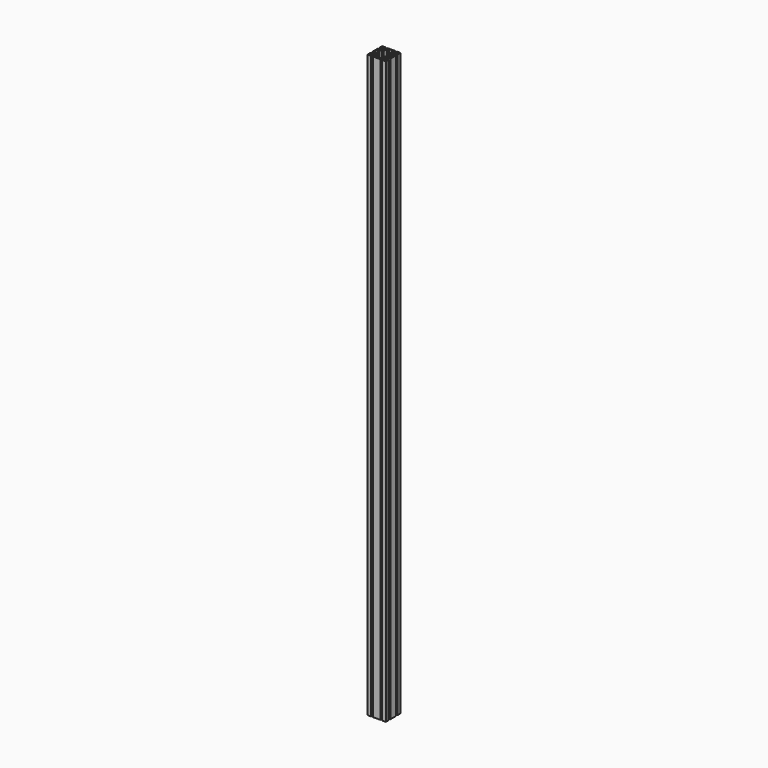
from build123d import *

# Parameters (mm, degrees)
F0_R     = 3
F0_R_2   = 2.5
F1_DEPTH = 1900
F2_R     = 2
F3_R     = 7


# Not quite as in the source:
# - a feature names something its author has since deleted; it is built from what else it names


with BuildPart() as f1:
    # F0 (on Top) → F1 (new body)
    with BuildSketch(Plane.XY):
        with BuildLine():
            Line((18.15, -30), (30, -30))
            Line((30, -30), (30, -18.15))
            Line((30, -18.15), (27.5, -18.15))
            Line((27.5, -18.15), (27.5, -20.15))
            Line((27.5, -20.15), (21.5477069044, -20.15))
            ThreePointArc((21.5477069044, -20.15), (19.5, -15), (21.5477069044, -9.85))
            Line((21.5477069044, -9.85), (27.5, -9.85))
            Line((27.5, -9.85), (27.5, -11.85))
            Line((27.5, -11.85), (30, -11.85))
            Line((30, -11.85), (30, 11.85))
            Line((30, 11.85), (27.5, 11.85))
            Line((27.5, 11.85), (27.5, 9.85))
            Line((27.5, 9.85), (21.5477069044, 9.85))
            ThreePointArc((21.5477069044, 9.85), (19.5, 15), (21.5477069044, 20.15))
            Line((21.5477069044, 20.15), (27.5, 20.15))
            Line((27.5, 20.15), (27.5, 18.15))
            Line((27.5, 18.15), (30, 18.15))
            Line((30, 18.15), (30, 30))
            Line((30, 30), (18.15, 30))
            Line((18.15, 30), (18.15, 27.5))
            Line((18.15, 27.5), (20.15, 27.5))
            Line((20.15, 27.5), (20.15, 21.5477069044))
            ThreePointArc((20.15, 21.5477069044), (15, 19.5), (9.85, 21.5477069044))
            Line((9.85, 21.5477069044), (9.85, 27.5))
            Line((9.85, 27.5), (11.85, 27.5))
            Line((11.85, 27.5), (11.85, 30))
            Line((11.85, 30), (-11.85, 30))
            Line((-11.85, 30), (-11.85, 27.5))
            Line((-11.85, 27.5), (-9.85, 27.5))
            Line((-9.85, 27.5), (-9.85, 21.5477069044))
            ThreePointArc((-9.85, 21.5477069044), (-15, 19.5), (-20.15, 21.5477069044))
            Line((-20.15, 21.5477069044), (-20.15, 27.5))
            Line((-20.15, 27.5), (-18.15, 27.5))
            Line((-18.15, 27.5), (-18.15, 30))
            Line((-18.15, 30), (-30, 30))
            Line((-30, 30), (-30, 18.15))
            Line((-30, 18.15), (-27.5, 18.15))
            Line((-27.5, 18.15), (-27.5, 20.15))
            Line((-27.5, 20.15), (-21.5477069044, 20.15))
            ThreePointArc((-21.5477069044, 20.15), (-19.5, 15), (-21.5477069044, 9.85))
            Line((-21.5477069044, 9.85), (-27.5, 9.85))
            Line((-27.5, 9.85), (-27.5, 11.85))
            Line((-27.5, 11.85), (-30, 11.85))
            Line((-30, 11.85), (-30, -11.85))
            Line((-30, -11.85), (-27.5, -11.85))
            Line((-27.5, -11.85), (-27.5, -9.85))
            Line((-27.5, -9.85), (-21.5477069044, -9.85))
            ThreePointArc((-21.5477069044, -9.85), (-19.5, -15), (-21.5477069044, -20.15))
            Line((-21.5477069044, -20.15), (-27.5, -20.15))
            Line((-27.5, -20.15), (-27.5, -18.15))
            Line((-27.5, -18.15), (-30, -18.15))
            Line((-30, -18.15), (-30, -30))
            Line((-30, -30), (-18.15, -30))
            Line((-18.15, -30), (-18.15, -27.5))
            Line((-18.15, -27.5), (-20.15, -27.5))
            Line((-20.15, -27.5), (-20.15, -21.5477069044))
            ThreePointArc((-20.15, -21.5477069044), (-15, -19.5), (-9.85, -21.5477069044))
            Line((-9.85, -21.5477069044), (-9.85, -27.5))
            Line((-9.85, -27.5), (-11.85, -27.5))
            Line((-11.85, -27.5), (-11.85, -30))
            Line((-11.85, -30), (11.85, -30))
            Line((11.85, -30), (11.85, -27.5))
            Line((11.85, -27.5), (9.85, -27.5))
            Line((9.85, -27.5), (9.85, -21.5477069044))
            ThreePointArc((9.85, -21.5477069044), (15, -19.5), (20.15, -21.5477069044))
            Line((20.15, -21.5477069044), (20.15, -27.5))
            Line((20.15, -27.5), (18.15, -27.5))
            Line((18.15, -27.5), (18.15, -30))
        make_face()
        with Locations((-25, -25)):
            Circle(F0_R, mode=Mode.SUBTRACT)
        with Locations((-15, -15)):
            Circle(F0_R_2, mode=Mode.SUBTRACT)
        with Locations((25, -25)):
            Circle(F0_R, mode=Mode.SUBTRACT)
        with Locations((15, -15)):
            Circle(F0_R_2, mode=Mode.SUBTRACT)
        with Locations((-25, 25)):
            Circle(F0_R, mode=Mode.SUBTRACT)
        with Locations((-15, 15)):
            Circle(F0_R_2, mode=Mode.SUBTRACT)
        Polygon((-7, 22), (-7, 27.5), (0, 27.5), (7, 27.5), (7, 22), (10, 16), (10, 10), (16, 10), (22, 7), (27.5, 7), (27.5, 0), (27.5, -7), (22, -7), (16, -10), (10, -10), (10, -16), (7, -22), (7, -27.5), (0, -27.5), (-7, -27.5), (-7, -22), (-10, -16), (-10, -10), (-16, -10), (-22, -7), (-27.5, -7), (-27.5, 0), (-27.5, 7), (-22, 7), (-16, 10), (-10, 10), (-10, 16), align=None, mode=Mode.SUBTRACT)
        with Locations((15, 15)):
            Circle(F0_R_2, mode=Mode.SUBTRACT)
        with Locations((25, 25)):
            Circle(F0_R, mode=Mode.SUBTRACT)
    extrude(amount=F1_DEPTH)

    # F2
    f2_edges = [f1.edges().sort_by_distance(p)[0] for p in [
        (-7, 27.5, 950),
        (7, 27.5, 950),
    ]]
    fillet(f2_edges, radius=F2_R)

    # F3
    f3_edges = [f1.edges().sort_by_distance(p)[0] for p in [
        (-10, 16, 950),
        (10, 16, 950),
    ]]
    fillet(f3_edges, radius=F3_R)


solid = f1.part
